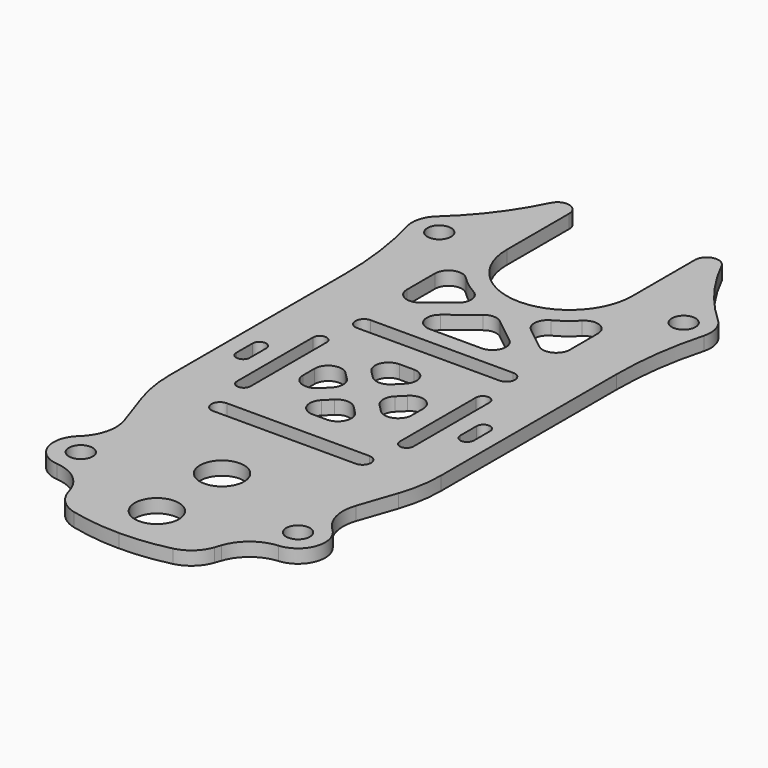
from build123d import *

# Parameters (mm, degrees)
F0_R     = 1.75
F0_R_2   = 3.25
F1_DEPTH = 2
F3_DEPTH = 25


# Not quite as in the source:
# - a feature names something its author has since deleted; it is built from what else it names


with BuildPart() as f1:
    # F0 (on Top) → F1 (new body)
    with BuildSketch(Plane.XY):
        with BuildLine():
            ThreePointArc((-12.5717246149, 50.2695334528), (-16.1191217808, 44.4802479149), (-20.6904345264, 39.4599935911))
            ThreePointArc((-20.6904345264, 39.4599935911), (-21.8414434806, 37.6150390062), (-21.8571428571, 35.4405430733))
            ThreePointArc((-21.8571428571, 35.4405430733), (-20.4663771338, 28.6163953155), (-20, 21.6676030258))
            Line((-20, 21.6676030258), (-20, -10.6856030045))
            ThreePointArc((-20, -10.6856030045), (-19.7308995433, -13.9554047127), (-18.9308396789, -17.1372159077))
            Line((-18.9308396789, -17.1372159077), (-17.0470641697, -22.6647409918))
            ThreePointArc((-17.0470641697, -22.6647409918), (-16.9162578432, -26.0979642803), (-18.6905264293, -29.0400899451))
            ThreePointArc((-18.6905264293, -29.0400899451), (-19.7861679358, -33.2903225806), (-16.3230484377, -35.9869336221))
            ThreePointArc((-16.3230484377, -35.9869336221), (-13.1213600073, -37.2332576723), (-11.1283691906, -40.0318501842))
            Line((-11.1283691906, -40.0318501842), (-10.837240035, -40.8861046865))
            ThreePointArc((-10.837240035, -40.8861046865), (-9.4747581102, -42.9666501557), (-7.2784782144, -44.1334325108))
            ThreePointArc((-7.2784782144, -44.1334325108), (-3.6649414842, -44.7825957956), (0, -45))
            ThreePointArc((0, -45), (3.6649414842, -44.7825957956), (7.2784782144, -44.1334325108))
            ThreePointArc((7.2784782144, -44.1334325108), (9.4747581102, -42.9666501557), (10.837240035, -40.8861046865))
            Line((10.837240035, -40.8861046865), (11.1283691906, -40.0318501842))
            ThreePointArc((11.1283691906, -40.0318501842), (13.1213600073, -37.2332576723), (16.3230484377, -35.9869336221))
            ThreePointArc((16.3230484377, -35.9869336221), (19.7861679358, -33.2903225806), (18.6905264293, -29.0400899451))
            ThreePointArc((18.6905264293, -29.0400899451), (16.9162578432, -26.0979642803), (17.0470641697, -22.6647409918))
            Line((17.0470641697, -22.6647409918), (18.9308396789, -17.1372159077))
            ThreePointArc((18.9308396789, -17.1372159077), (19.7308995433, -13.9554047127), (20, -10.6856030045))
            Line((20, -10.6856030045), (20, 21.6676030258))
            ThreePointArc((20, 21.6676030258), (20.4663771338, 28.6163953155), (21.8571428571, 35.4405430733))
            ThreePointArc((21.8571428571, 35.4405430733), (21.8414434806, 37.6150390062), (20.6904345264, 39.4599935911))
            ThreePointArc((20.6904345264, 39.4599935911), (16.1191217808, 44.4802479149), (12.5717246149, 50.2695334528))
            ThreePointArc((12.5717246149, 50.2695334528), (10.6050430884, 51.2048486848), (9.25, 49.5))
            Line((9.25, 49.5), (9.25, 38))
            ThreePointArc((9.25, 38), (0, 28.75), (-9.25, 38))
            Line((-9.25, 38), (-9.25, 49.5))
            ThreePointArc((-9.25, 49.5), (-10.6050430884, 51.2048486848), (-12.5717246149, 50.2695334528))
        make_face()
        with Locations((-16, -32)):
            Circle(F0_R, mode=Mode.SUBTRACT)
        with BuildLine():
            Line((-17.5, -1.5), (-17.5, 1.5))
            ThreePointArc((-17.5, 1.5), (-16.5, 2.5), (-15.5, 1.5))
            Line((-15.5, 1.5), (-15.5, -1.5))
            ThreePointArc((-15.5, -1.5), (-16.5, -2.5), (-17.5, -1.5))
        make_face(mode=Mode.SUBTRACT)
        with BuildLine():
            Line((-13, -7), (-13, 7))
            ThreePointArc((-13, 7), (-12, 8), (-11, 7))
            Line((-11, 7), (-11, -7))
            ThreePointArc((-11, -7), (-12, -8), (-13, -7))
        make_face(mode=Mode.SUBTRACT)
        with Locations((0, -38)):
            Circle(F0_R_2, mode=Mode.SUBTRACT)
        with Locations((0, -26)):
            Circle(F0_R_2, mode=Mode.SUBTRACT)
        with Locations((16, -32)):
            Circle(F0_R, mode=Mode.SUBTRACT)
        with BuildLine():
            Line((10.5, -14.5), (-10.5, -14.5))
            ThreePointArc((-10.5, -14.5), (-11.75, -13.25), (-10.5, -12))
            Line((-10.5, -12), (10.5, -12))
            ThreePointArc((10.5, -12), (11.75, -13.25), (10.5, -14.5))
        make_face(mode=Mode.SUBTRACT)
        with BuildLine():
            Line((11, -7), (11, 7))
            ThreePointArc((11, 7), (12, 8), (13, 7))
            Line((13, 7), (13, -7))
            ThreePointArc((13, -7), (12, -8), (11, -7))
        make_face(mode=Mode.SUBTRACT)
        with BuildLine():
            Line((15.5, -1.5), (15.5, 1.5))
            ThreePointArc((15.5, 1.5), (16.5, 2.5), (17.5, 1.5))
            Line((17.5, 1.5), (17.5, -1.5))
            ThreePointArc((17.5, -1.5), (16.5, -2.5), (15.5, -1.5))
        make_face(mode=Mode.SUBTRACT)
        with Locations((-18, 36.5)):
            Circle(F0_R, mode=Mode.SUBTRACT)
        with BuildLine():
            Line((10.5, 12), (-10.5, 12))
            ThreePointArc((-10.5, 12), (-11.75, 13.25), (-10.5, 14.5))
            Line((-10.5, 14.5), (10.5, 14.5))
            ThreePointArc((10.5, 14.5), (11.75, 13.25), (10.5, 12))
        make_face(mode=Mode.SUBTRACT)
        with Locations((18, 36.5)):
            Circle(F0_R, mode=Mode.SUBTRACT)
    extrude(amount=F1_DEPTH)

    # F2 (on face) → F3 (cut)
    with BuildSketch(Plane.XY.offset(2)):
        with BuildLine():
            Line((1.0502525317, 8), (-1.0502525317, 8))
            ThreePointArc((-1.0502525317, 8), (-2.8980115967, 6.7653668647), (-2.4644660941, 4.5857864376))
            Line((-2.4644660941, 4.5857864376), (-1.4142135624, 3.5355339059))
            ThreePointArc((-1.4142135624, 3.5355339059), (0, 2.9497474683), (1.4142135624, 3.5355339059))
            Line((1.4142135624, 3.5355339059), (2.4644660941, 4.5857864376))
            ThreePointArc((2.4644660941, 4.5857864376), (2.8980115967, 6.7653668647), (1.0502525317, 8))
        make_face()
        with BuildLine():
            ThreePointArc((-2.4644660941, -4.5857864376), (-2.8980115967, -6.7653668647), (-1.0502525317, -8))
            Line((-1.0502525317, -8), (1.0502525317, -8))
            ThreePointArc((1.0502525317, -8), (2.8980115967, -6.7653668647), (2.4644660941, -4.5857864376))
            Line((2.4644660941, -4.5857864376), (1.4142135624, -3.5355339059))
            ThreePointArc((1.4142135624, -3.5355339059), (0, -2.9497474683), (-1.4142135624, -3.5355339059))
            Line((-1.4142135624, -3.5355339059), (-2.4644660941, -4.5857864376))
        make_face()
        with BuildLine():
            ThreePointArc((-4.5857864376, 2.4644660941), (-6.7653668647, 2.8980115967), (-8, 1.0502525317))
            Line((-8, 1.0502525317), (-8, -1.0502525317))
            ThreePointArc((-8, -1.0502525317), (-6.7653668647, -2.8980115967), (-4.5857864376, -2.4644660941))
            Line((-4.5857864376, -2.4644660941), (-3.5355339059, -1.4142135624))
            ThreePointArc((-3.5355339059, -1.4142135624), (-2.9497474683, 0), (-3.5355339059, 1.4142135624))
            Line((-3.5355339059, 1.4142135624), (-4.5857864376, 2.4644660941))
        make_face()
        with BuildLine():
            Line((8, -1.0502525317), (8, 1.0502525317))
            ThreePointArc((8, 1.0502525317), (6.7653668647, 2.8980115967), (4.5857864376, 2.4644660941))
            Line((4.5857864376, 2.4644660941), (3.5355339059, 1.4142135624))
            ThreePointArc((3.5355339059, 1.4142135624), (2.9497474683, 0), (3.5355339059, -1.4142135624))
            Line((3.5355339059, -1.4142135624), (4.5857864376, -2.4644660941))
            ThreePointArc((4.5857864376, -2.4644660941), (6.7653668647, -2.8980115967), (8, -1.0502525317))
        make_face()
        with BuildLine():
            ThreePointArc((-5.0763219385, 20.5680916489), (-5.7238553417, 18.3428026544), (-3.8349160497, 17))
            Line((-3.8349160497, 17), (3.8349160497, 17))
            ThreePointArc((3.8349160497, 17), (5.7238553417, 18.3428026544), (5.0763219385, 20.5680916489))
            Line((5.0763219385, 20.5680916489), (1.2414058887, 23.604066855))
            ThreePointArc((1.2414058887, 23.604066855), (0, 24.035975206), (-1.2414058887, 23.604066855))
            Line((-1.2414058887, 23.604066855), (-5.0763219385, 20.5680916489))
        make_face()
        with BuildLine():
            ThreePointArc((-8.5714285714, 29.6017494533), (-10.755928946, 30.0536812284), (-12, 28.2020410289))
            Line((-12, 28.2020410289), (-12, 23.0473581273))
            ThreePointArc((-12, 23.0473581273), (-10.870973083, 21.246967645), (-8.7585941113, 21.4792664784))
            Line((-8.7585941113, 21.4792664784), (-5.4230382746, 24.1199148491))
            ThreePointArc((-5.4230382746, 24.1199148491), (-4.6719651901, 25.8612910654), (-5.7123807114, 27.4468627126))
            ThreePointArc((-5.7123807114, 27.4468627126), (-7.2227201333, 28.4170821836), (-8.5714285714, 29.6017494533))
        make_face()
        with BuildLine():
            Line((12, 23.0473581273), (12, 28.2020410289))
            ThreePointArc((12, 28.2020410289), (10.755928946, 30.0536812284), (8.5714285714, 29.6017494533))
            ThreePointArc((8.5714285714, 29.6017494533), (7.2227201333, 28.4170821836), (5.7123807114, 27.4468627126))
            ThreePointArc((5.7123807114, 27.4468627126), (4.6719651901, 25.8612910654), (5.4230382746, 24.1199148491))
            Line((5.4230382746, 24.1199148491), (8.7585941113, 21.4792664784))
            ThreePointArc((8.7585941113, 21.4792664784), (10.870973083, 21.246967645), (12, 23.0473581273))
        make_face()
    extrude(amount=-F3_DEPTH, mode=Mode.SUBTRACT)


solid = f1.part
